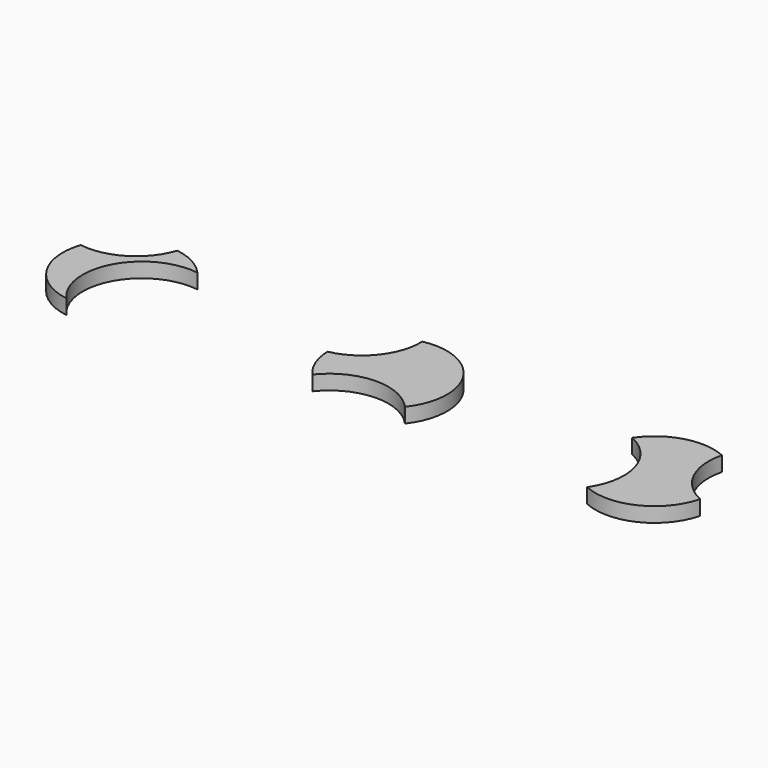
from build123d import *

# Parameters (mm, degrees)
F1_DEPTH = 1.5875


# Not quite as in the source:
# - a feature of the source that left no trace in its solid (it failed there, or was rolled back) is left out


with BuildPart() as f1:
    # F0 (on Top) → F1 (new body, symmetric)
    with BuildSketch(Plane.XY):
        with BuildLine():
            ThreePointArc((28.2155579418, 7.1429440823), (35.2262329925, -0.9860169952), (33.5054625888, -11.5817011206))
            ThreePointArc((33.5054625888, -11.5817011206), (44.2389831087, -11.4364079158), (51.0270560551, -3.1206614946))
            ThreePointArc((51.0270560551, -3.1206614946), (44.8016172576, 2.9384882245), (43.9274008255, 11.5817011206))
            ThreePointArc((43.9274008255, 11.5817011206), (35.2636916641, 12.2216441691), (28.2155579418, 7.1429440823))
        make_face()
    extrude(amount=F1_DEPTH, both=True)


with BuildPart() as f1b:
    # F0 (on Top) → F1, piece 2 (new body, symmetric)
    with BuildSketch(Plane.XY):
        with BuildLine():
            ThreePointArc((-87.7515485228, 4.0306815011), (-86.5371761619, -6.634911433), (-77.5862744551, -12.5603592221))
            ThreePointArc((-77.5862744551, -12.5603592221), (-79.234417553, 1.9149565428), (-66.1957682837, 8.4145540225))
            ThreePointArc((-66.1957682837, 8.4145540225), (-69.6473816706, 11.1605182273), (-73.830012371, 12.5603592221))
            ThreePointArc((-73.830012371, 12.5603592221), (-79.2385060477, 5.7620079744), (-87.7515485228, 4.0306815011))
        make_face()
    extrude(amount=F1_DEPTH, both=True)


with BuildPart() as f1c:
    # F0 (on Top) → F1, piece 3 (new body, symmetric)
    with BuildSketch(Plane.XY):
        with BuildLine():
            ThreePointArc((-28.0400193697, -8.4381200139), (-18.444887024, -3.6253237231), (-8.5904389845, -7.8820157138))
            ThreePointArc((-8.5904389845, -7.8820157138), (-7.7359985931, 6.661748372), (-21.1104305579, 12.4389199798))
            ThreePointArc((-21.1104305579, 12.4389199798), (-23.8471389134, 4.1939329625), (-31.2433546383, -0.3629713035))
            ThreePointArc((-31.2433546383, -0.3629713035), (-30.3536202994, -4.6829628767), (-28.0400193697, -8.4381200139))
        make_face()
    extrude(amount=F1_DEPTH, both=True)


solid = Compound([f1.part, f1b.part, f1c.part])
